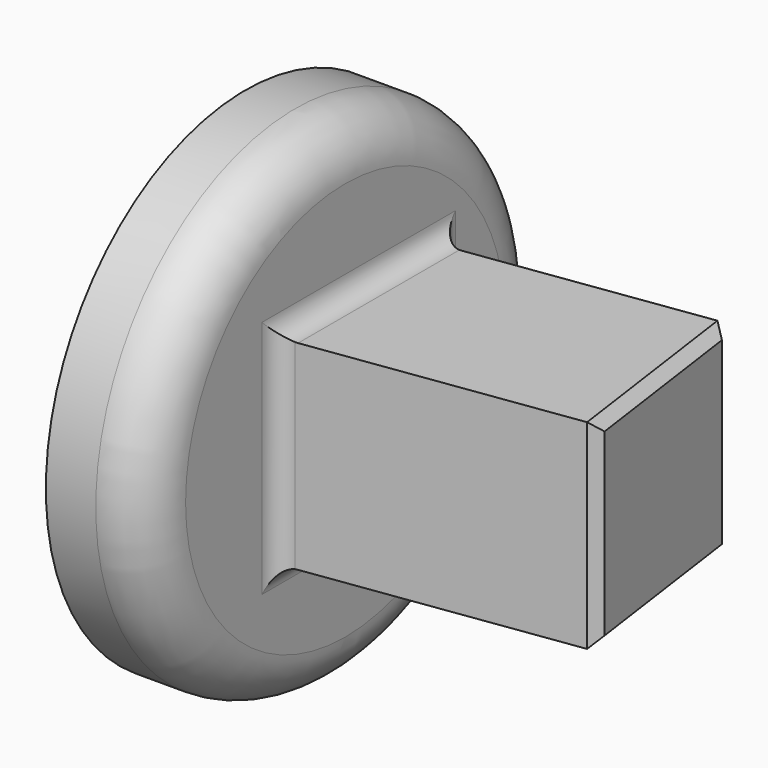
from build123d import *

# Parameters (mm, degrees)
F0_R     = 25
F1_DEPTH = 10
F5_W     = 20
F5_H     = 20
F6_DEPTH = 31
F7_SIZE  = 1
F8_R     = 5
F9_R     = 2


# Not quite as in the source:
# - a feature names something its author has since deleted; it is built from what else it names


with BuildPart() as f1:
    # F0 (on Right) → F1 (new body)
    with BuildSketch(Plane.YZ):
        Circle(F0_R)
    extrude(amount=F1_DEPTH)

    # F5 (on offset) → F6 (join)
    with BuildSketch(Plane(origin=(6.9318764812, 0.9742117067, 0), x_dir=(0.139173101, -0.9902680687, 0), z_dir=(-0.9902680687, -0.139173101, 0))):
        Rectangle(F5_W, F5_H)
    extrude(amount=-F6_DEPTH)

    # F7
    f7_edges = [f1.edges().sort_by_distance(p)[0] for p in [
        (39.021918, -4.614103, 0),
        (37.630187, 5.288578, 10),
        (36.238456, 15.191259, 0),
        (37.630187, 5.288578, -10),
    ]]
    chamfer(f7_edges, length=F7_SIZE)

    # F8
    f8_edges = [f1.edges().sort_by_distance(p)[0] for p in [
        (10, -25, 0),
    ]]
    fillet(f8_edges, radius=F8_R)

    # F9
    f9_edges = [f1.edges().sort_by_distance(p)[0] for p in [
        (10, 1.405408, -10),
        (10, -8.692867, 0),
        (10, 1.405408, 10),
        (10, 11.503684, 0),
    ]]
    fillet(f9_edges, radius=F9_R)


solid = f1.part
